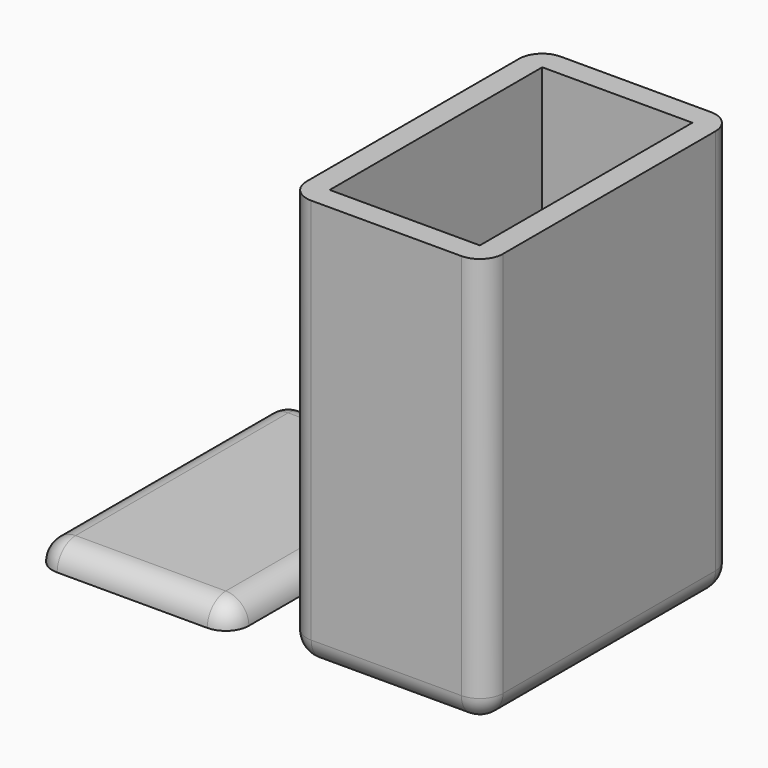
from build123d import *

# Parameters (mm, degrees)
F0_W     = 17
F0_H     = 27
F1_DEPTH = 35.5
F2_W     = 13
F2_H     = 23
F3_DEPTH = 33.5
F4_R     = 2
F6_DEPTH = 2
F7_R     = 1.99999


# Not quite as in the source:
# - a fillet or chamfer is up to 0.001 mm smaller than in the source, because OpenCascade refuses the exact size


with BuildPart() as f1:
    # F0 (on Top) → F1 (new body)
    with BuildSketch(Plane.XY):
        with Locations((8.5, 13.5)):
            Rectangle(F0_W, F0_H)
    extrude(amount=F1_DEPTH)

    # F2 (on face) → F3 (cut)
    with BuildSketch(Plane.XY.offset(35.5)):
        with Locations((8.5, 13.5)):
            Rectangle(F2_W, F2_H)
    extrude(amount=-F3_DEPTH, mode=Mode.SUBTRACT)

    # F4
    f4_edges = [f1.edges().sort_by_distance(p)[0] for p in [
        (0, 13.5, 0),
        (8.5, 0, 0),
        (17, 13.5, 0),
        (8.5, 27, 0),
        (17, 0, 17.75),
        (0, 0, 17.75),
        (17, 27, 17.75),
        (0, 27, 17.75),
    ]]
    fillet(f4_edges, radius=F4_R)


with BuildPart() as f6:
    # F5 (on Top) → F6 (new body)
    with BuildSketch(Plane.XY):
        with BuildLine():
            Line((-20, 0), (-7, 0))
            ThreePointArc((-7, 0), (-5.5857864376, 0.5857864376), (-5, 2))
            Line((-5, 2), (-5, 25))
            ThreePointArc((-5, 25), (-5.5857864376, 26.4142135624), (-7, 27))
            Line((-7, 27), (-20, 27))
            ThreePointArc((-20, 27), (-21.4142135624, 26.4142135624), (-22, 25))
            Line((-22, 25), (-22, 2))
            ThreePointArc((-22, 2), (-21.4142135624, 0.5857864376), (-20, 0))
        make_face()
    extrude(amount=F6_DEPTH)

    # F7 (radius 2 in the source; OpenCascade refuses exactly that, so slightly less here)
    f7_edges = [f6.edges().sort_by_distance(p)[0] for p in [
        (-13.5, 0, 2),
        (-5.585786, 0.585786, 2),
        (-5, 13.5, 2),
        (-5.585786, 26.414214, 2),
        (-13.5, 27, 2),
        (-21.414214, 26.414214, 2),
        (-22, 13.5, 2),
        (-21.414214, 0.585786, 2),
    ]]
    fillet(f7_edges, radius=F7_R)


solid = Compound([f1.part, f6.part])
